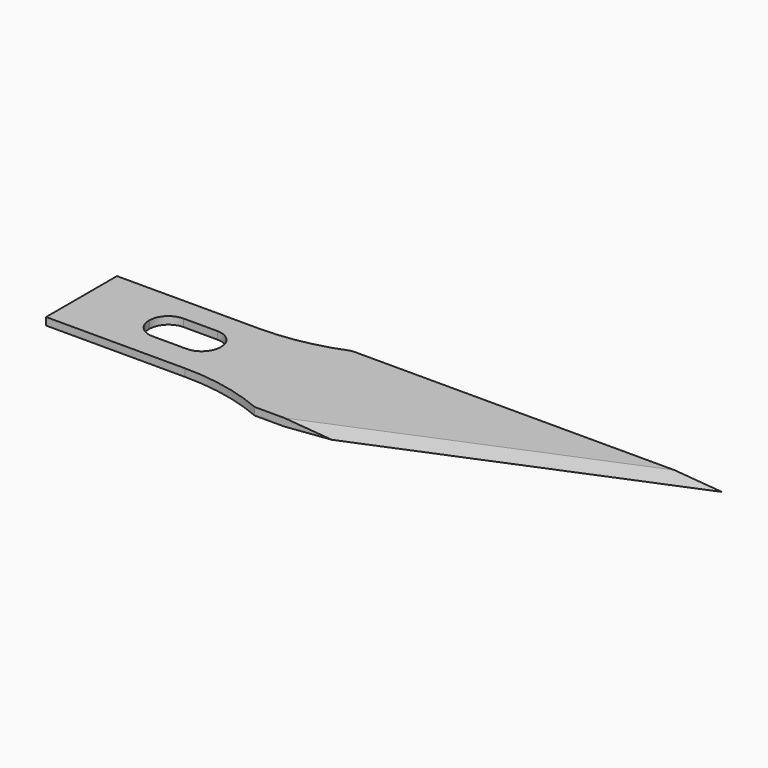
from build123d import *

# Parameters (mm, degrees)
F1_DEPTH    = 0.5
F2_T1_DEPTH = 0.5
F3_W        = 4.74
F3_H        = 2.55
F4_DEPTH    = 0.501
F5_R        = 1.25
F6_SIZE2    = 1.19999
F6_SIZE     = 0.24999


# Not quite as in the source:
# - a fillet or chamfer that OpenCascade refuses, or shapes differently, is made with other operations: its cross-section is extruded or revolved along the edge and cut away or added
# - a fillet or chamfer is up to 0.001 mm smaller than in the source, because OpenCascade refuses the exact size


with BuildPart() as f1:
    # F0 (on Top) → F1 (new body)
    with BuildSketch(Plane.XY):
        Polygon((0, 5.86), (0, 0), (14.7, 0), (14.7, -1.13), (19.8, -1.13), (39.17, 6.9), (14.7, 6.9), (14.7, 5.86), align=None)
    extrude(amount=F1_DEPTH)

    # F2: fillet of radius 14 on 2 edges, made by hand

    # F2_s2 → F2_t1 (join)
    with BuildSketch(Plane.XY):
        with BuildLine():
            ThreePointArc((14.7, 6.9), (12.1030176748, 6.1224601911), (9.4048701621, 5.86))
            Line((9.4048701621, 5.86), (14.7, 5.86))
            Line((14.7, 5.86), (14.7, 6.9))
        make_face()
        with BuildLine():
            ThreePointArc((9.1897277744, 0), (12.0021999965, -0.2854092296), (14.7, -1.13))
            Line((14.7, -1.13), (14.7, 0))
            Line((14.7, 0), (9.1897277744, 0))
        make_face()
    extrude(amount=F2_T1_DEPTH)

    # F3 (on face) → F4 (cut, through all)
    with BuildSketch(Plane.XY.offset(0.5)):
        with Locations((6.77, 3.025)):
            Rectangle(F3_W, F3_H)
    extrude(amount=-F4_DEPTH, mode=Mode.SUBTRACT)

    # F5
    f5_edges = [f1.edges().sort_by_distance(p)[0] for p in [
        (9.14, 1.75, 0.25),
        (4.4, 1.75, 0.25),
        (4.4, 4.3, 0.25),
        (9.14, 4.3, 0.25),
    ]]
    fillet(f5_edges, radius=F5_R)

    # F6 (size 0.25 and 1.2 in the source; OpenCascade refuses exactly that, so slightly less here)
    f6_edges = [f1.edges().sort_by_distance(p)[0] for p in [
        (29.485, 2.885, 0.5),
        (29.485, 2.885, 0),
    ]]
    f6_side = f1.faces().sort_by_distance((29.485, 2.885, 0.25))[0]
    chamfer(f6_edges, length=F6_SIZE, length2=F6_SIZE2, reference=f6_side)


solid = f1.part
